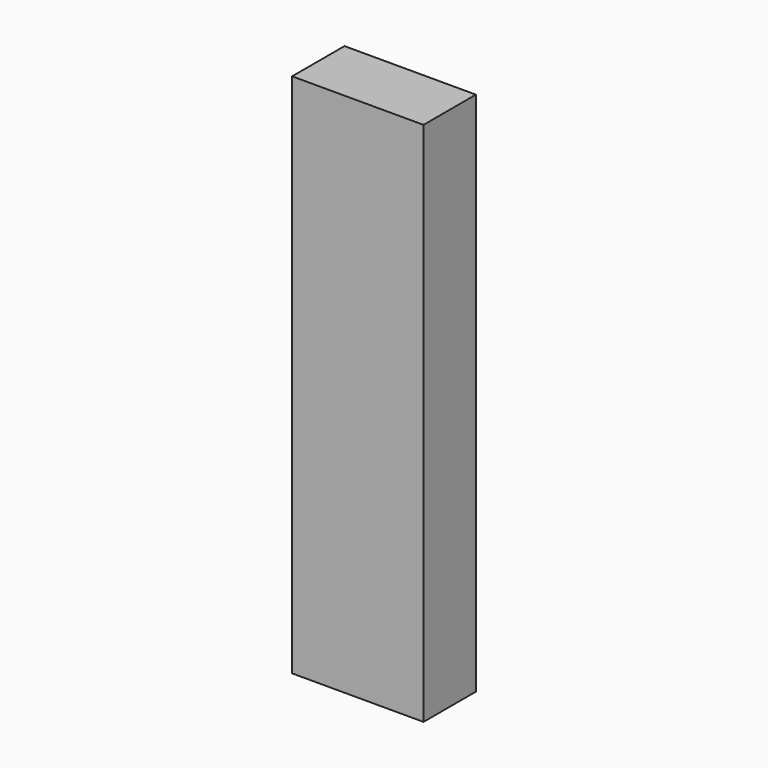
from build123d import *

# Parameters (mm, degrees)
F0_W     = 25.4947114736
F0_H     = 43.1240350008
F1_DEPTH = 25.4
F2_T     = -2.54
F4_W     = 12.7473566681
F4_H     = 50.9894266725
F5_DEPTH = 6.35


with BuildPart() as f1:
    # F0 (on Front) → F1 (new body)
    with BuildSketch(Plane.XZ):
        with Locations((12.7473557368, 21.5620175004)):
            Rectangle(F0_W, F0_H)
    extrude(amount=F1_DEPTH)

    # F2
    f2_openings = [f1.faces().sort_by_distance(p)[0] for p in [
        (12.747356, -12.7, 43.124035),
    ]]
    offset(amount=F2_T, openings=f2_openings)


with BuildPart() as f5:
    # F4 (on Front) → F5 (new body)
    with BuildSketch(Plane.XZ):
        with Locations((-6.3736783341, 25.4947133362)):
            Rectangle(F4_W, F4_H)
    extrude(amount=F5_DEPTH)


solid = f5.part
